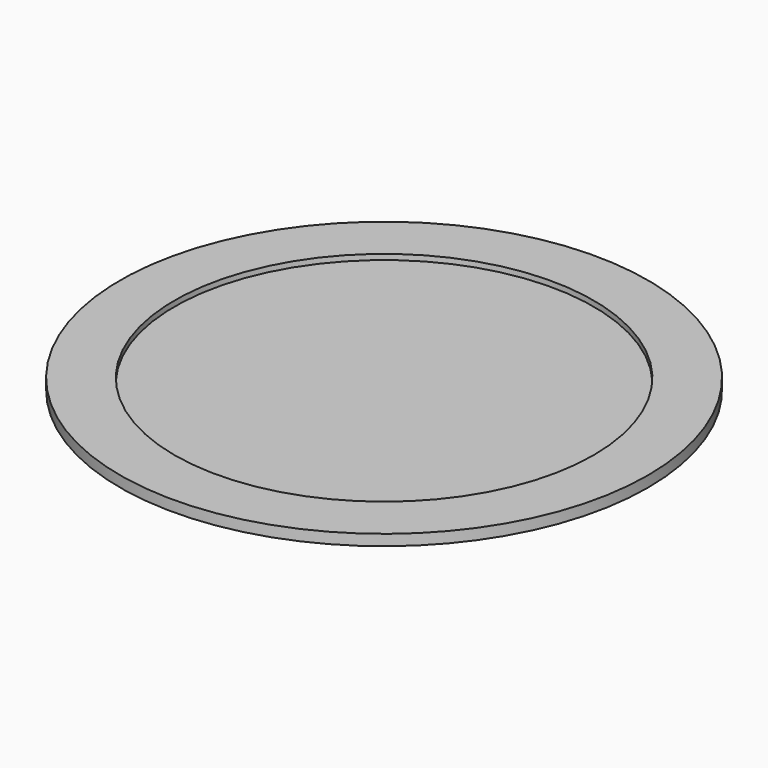
from build123d import *

# Parameters (mm, degrees)
F0_R     = 48.5
F1_DEPTH = 2
F4_R     = 38.5
F5_DEPTH = 1


with BuildPart() as f1:
    # F0 (on Top) → F1 (new body)
    with BuildSketch(Plane.XY):
        Circle(F0_R)
    extrude(amount=F1_DEPTH)

    # F4 (on face) → F5 (cut)
    with BuildSketch(Plane.XY.offset(2)):
        Circle(F4_R)
    extrude(amount=-F5_DEPTH, mode=Mode.SUBTRACT)


solid = f1.part
